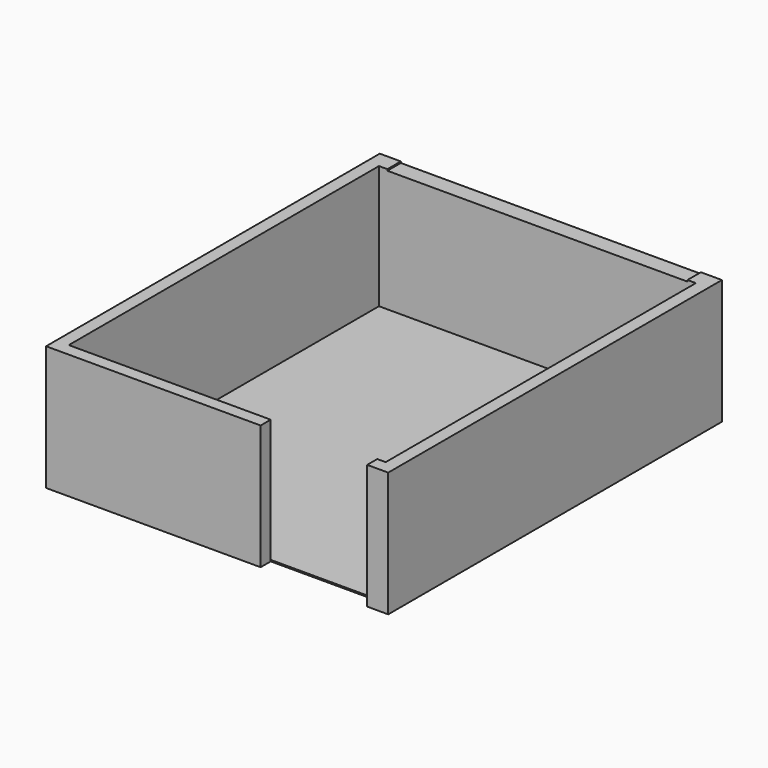
from build123d import *

# Parameters (mm, degrees)
F0_W        = 2717.8
F0_H        = 152.4000000021
F0_W_2      = 965.2
F0_H_2      = 114.3
F1_DEPTH    = 1117.6
F1_FACE_W   = 3098.8
F1_FACE_H   = 3778.2500000021
F1_FACE_W_2 = 2870.2
F1_FACE_H_2 = 3511.55
F2_DEPTH    = 12.7
F3_DEPTH    = 2387.6
F4_DEPTH    = 1117.6
F5_DEPTH    = 2159


# Not quite as in the source:
# - a feature names something its author has since deleted; it is built from what else it names


with BuildPart() as f1:
    # F0 (on Top) → F1 (new body)
    with BuildSketch(Plane.XY):
        Polygon((190.5, 3778.2500000021), (0, 3778.2500000021), (0, 0), (1943.1, 0), (1943.1, 114.3), (114.3, 114.3), (114.3, 3625.85), (190.5, 3625.85), align=None)
        with Locations((1549.4, 3702.050000001)):
            Rectangle(F0_W, F0_H)
        Polygon((3098.8, 3778.2500000021), (2908.3, 3778.2500000021), (2908.3, 3625.85), (2984.5, 3625.85), (2984.5, 114.3), (2908.3, 114.3), (2908.3, 0), (3098.8, 0), align=None)
        with Locations((2425.7, 57.15)):
            Rectangle(F0_W_2, F0_H_2)
    extrude(amount=F1_DEPTH)

    # F0 (on Top) + F1_face (on face) → F2 (join)
    with BuildSketch(Plane.XY):
        Polygon((2908.3, 3625.85), (190.5, 3625.85), (114.3, 3625.85), (114.3, 114.3), (1943.1, 114.3), (2908.3, 114.3), (2984.5, 114.3), (2984.5, 3625.85), align=None)
    with BuildSketch(Plane(origin=(1549.4, 2006.9762474082, 1117.6), x_dir=(1, 0, 0), z_dir=(0, 0, 1))):
        with Locations((0, -117.8512474072)):
            Rectangle(F1_FACE_W, F1_FACE_H)
        with Locations((0, -136.9012474082)):
            Rectangle(F1_FACE_W_2, F1_FACE_H_2, mode=Mode.SUBTRACT)
    extrude(amount=F2_DEPTH)

    # F0 (on Top) → F3 (cut)
    with BuildSketch(Plane.XY):
        with Locations((1549.4, 3702.050000001)):
            Rectangle(F0_W, F0_H)
    extrude(amount=F3_DEPTH, mode=Mode.SUBTRACT)

    # F0 (on Top) → F4 (join)
    with BuildSketch(Plane.XY):
        with Locations((1549.4, 3702.050000001)):
            Rectangle(F0_W, F0_H)
    extrude(amount=F4_DEPTH)

    # F0 (on Top) → F5 (cut)
    with BuildSketch(Plane.XY):
        with Locations((2425.7, 57.15)):
            Rectangle(F0_W_2, F0_H_2)
    extrude(amount=F5_DEPTH, mode=Mode.SUBTRACT)


solid = f1.part
